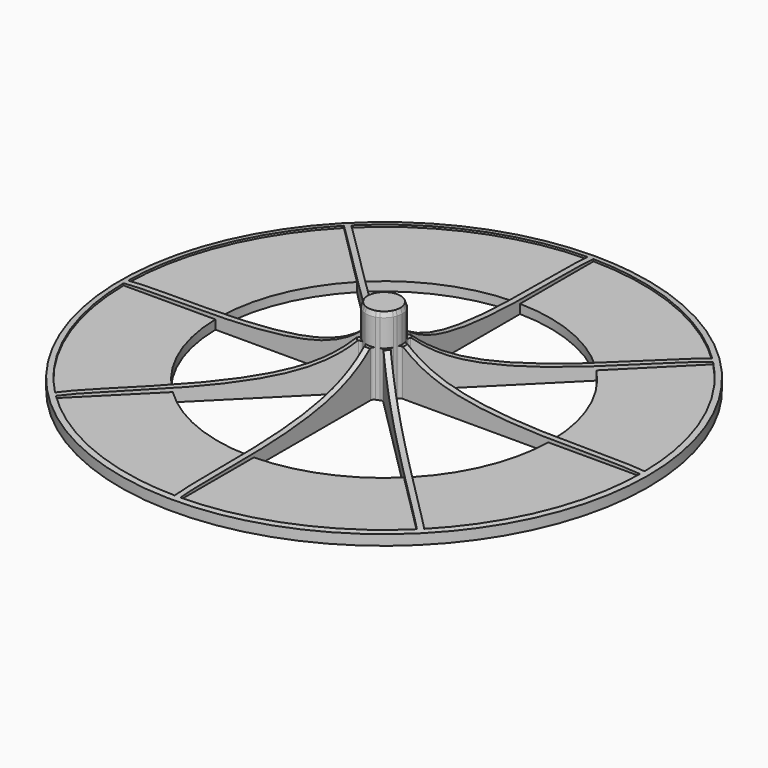
from build123d import *

# Parameters (mm, degrees)
F0_R     = 58.42
F1_DEPTH = 10.16
F2_R     = 58.42
F2_R_2   = 36.83
F3_DEPTH = 2
F7_DEPTH = 7
F8_SIZE2 = 1.0467888968
F8_SIZE  = 0.381


# Not quite as in the source:
# - a feature names something its author has since deleted; it is built from what else it names


with BuildPart() as f1:
    # F0 (on Top) → F1 (new body)
    with BuildSketch(Plane.XY):
        Circle(F0_R)
        with BuildLine():
            ThreePointArc((-0.635, -57.1464721133), (-21.8703581597, -52.799715283), (-39.9596451462, -40.8576707583))
            Line((-39.9596451462, -40.8576707583), (-27.3861598627, -28.2841854748))
            Line((-27.3861598627, -28.2841854748), (-2.7700736327, -3.6680992448))
            ThreePointArc((-2.7700736327, -3.6680992448), (-2.3442801324, -3.4533430776), (-1.8742194586, -3.5337375994))
            ThreePointArc((-1.8742194586, -3.5337375994), (-1.5307337295, -3.69551813), (-1.1734565309, -3.824003108))
            ThreePointArc((-1.1734565309, -3.824003108), (-0.7842259293, -4.0995386865), (-0.635, -4.5524757001))
            Line((-0.635, -4.5524757001), (-0.635, -38.0947079658))
            Line((-0.635, -38.0947079658), (-0.635, -57.1464721133))
        make_face(mode=Mode.SUBTRACT)
        with BuildLine():
            ThreePointArc((-40.8576707583, -39.9596451462), (-52.799715283, -21.8703581597), (-57.1464721133, -0.635))
            Line((-57.1464721133, -0.635), (-39.3648786992, -0.635))
            Line((-39.3648786992, -0.635), (-4.5524757001, -0.635))
            ThreePointArc((-4.5524757001, -0.635), (-4.0995386865, -0.7842259293), (-3.824003108, -1.1734565309))
            ThreePointArc((-3.824003108, -1.1734565309), (-3.69551813, -1.5307337295), (-3.5337375994, -1.8742194586))
            ThreePointArc((-3.5337375994, -1.8742194586), (-3.4533430776, -2.3442801324), (-3.6680992448, -2.7700736327))
            Line((-3.6680992448, -2.7700736327), (-27.386039136, -26.4880135239))
            Line((-27.386039136, -26.4880135239), (-40.8576707583, -39.9596451462))
        make_face(mode=Mode.SUBTRACT)
        with BuildLine():
            ThreePointArc((39.9596451462, -40.8576707583), (21.8703581597, -52.799715283), (0.635, -57.1464721133))
            Line((0.635, -57.1464721133), (0.635, -39.3648786992))
            Line((0.635, -39.3648786992), (0.635, -4.5524757001))
            ThreePointArc((0.635, -4.5524757001), (0.7842259293, -4.0995386865), (1.1734565309, -3.824003108))
            ThreePointArc((1.1734565309, -3.824003108), (1.5307337295, -3.69551813), (1.8742194586, -3.5337375994))
            ThreePointArc((1.8742194586, -3.5337375994), (2.3442801324, -3.4533430776), (2.7700736327, -3.6680992448))
            Line((2.7700736327, -3.6680992448), (27.3861598627, -28.2841854748))
            Line((27.3861598627, -28.2841854748), (39.9596451462, -40.8576707583))
        make_face(mode=Mode.SUBTRACT)
        with BuildLine():
            ThreePointArc((57.1464721133, -0.635), (52.799715283, -21.8703581597), (40.8576707583, -39.9596451462))
            Line((40.8576707583, -39.9596451462), (27.386039136, -26.4880135239))
            Line((27.386039136, -26.4880135239), (3.6680992448, -2.7700736327))
            ThreePointArc((3.6680992448, -2.7700736327), (3.4533430776, -2.3442801324), (3.5337375994, -1.8742194586))
            ThreePointArc((3.5337375994, -1.8742194586), (3.69551813, -1.5307337295), (3.824003108, -1.1734565309))
            ThreePointArc((3.824003108, -1.1734565309), (4.0995386865, -0.7842259293), (4.5524757001, -0.635))
            Line((4.5524757001, -0.635), (38.0947079658, -0.635))
            Line((38.0947079658, -0.635), (57.1464721133, -0.635))
        make_face(mode=Mode.SUBTRACT)
        with BuildLine():
            ThreePointArc((-3.6680992448, 2.7700736327), (-3.4533430776, 2.3442801324), (-3.5337375994, 1.8742194586))
            ThreePointArc((-3.5337375994, 1.8742194586), (-3.69551813, 1.5307337295), (-3.824003108, 1.1734565309))
            ThreePointArc((-3.824003108, 1.1734565309), (-4.0995386865, 0.7842259293), (-4.5524757001, 0.635))
            Line((-4.5524757001, 0.635), (-38.0947079658, 0.635))
            Line((-38.0947079658, 0.635), (-57.1464721133, 0.635))
            ThreePointArc((-57.1464721133, 0.635), (-52.799715283, 21.8703581597), (-40.8576707583, 39.9596451462))
            Line((-40.8576707583, 39.9596451462), (-27.386039136, 26.4880135239))
            Line((-27.386039136, 26.4880135239), (-3.6680992448, 2.7700736327))
        make_face(mode=Mode.SUBTRACT)
        with BuildLine():
            ThreePointArc((-39.9596451462, 40.8576707583), (-21.8703581597, 52.799715283), (-0.635, 57.1464721133))
            Line((-0.635, 57.1464721133), (-0.635, 39.3648786992))
            Line((-0.635, 39.3648786992), (-0.635, 4.5524757001))
            ThreePointArc((-0.635, 4.5524757001), (-0.7842259293, 4.0995386865), (-1.1734565309, 3.824003108))
            ThreePointArc((-1.1734565309, 3.824003108), (-1.5307337295, 3.69551813), (-1.8742194586, 3.5337375994))
            ThreePointArc((-1.8742194586, 3.5337375994), (-2.3442801324, 3.4533430776), (-2.7700736327, 3.6680992448))
            Line((-2.7700736327, 3.6680992448), (-26.4880135239, 27.386039136))
            Line((-26.4880135239, 27.386039136), (-39.9596451462, 40.8576707583))
        make_face(mode=Mode.SUBTRACT)
        with BuildLine():
            ThreePointArc((40.8576707583, 39.9596451462), (52.799715283, 21.8703581597), (57.1464721133, 0.635))
            Line((57.1464721133, 0.635), (39.3648786992, 0.635))
            Line((39.3648786992, 0.635), (4.5524757001, 0.635))
            ThreePointArc((4.5524757001, 0.635), (4.0995386865, 0.7842259293), (3.824003108, 1.1734565309))
            ThreePointArc((3.824003108, 1.1734565309), (3.69551813, 1.5307337295), (3.5337375994, 1.8742194586))
            ThreePointArc((3.5337375994, 1.8742194586), (3.4533430776, 2.3442801324), (3.6680992448, 2.7700736327))
            Line((3.6680992448, 2.7700736327), (28.2841854748, 27.3861598627))
            Line((28.2841854748, 27.3861598627), (40.8576707583, 39.9596451462))
        make_face(mode=Mode.SUBTRACT)
        with BuildLine():
            Line((0.635, 38.0947079658), (0.635, 57.1464721133))
            ThreePointArc((0.635, 57.1464721133), (21.8703581597, 52.799715283), (39.9596451462, 40.8576707583))
            Line((39.9596451462, 40.8576707583), (26.4880135239, 27.386039136))
            Line((26.4880135239, 27.386039136), (2.7700736327, 3.6680992448))
            ThreePointArc((2.7700736327, 3.6680992448), (2.3442801324, 3.4533430776), (1.8742194586, 3.5337375994))
            ThreePointArc((1.8742194586, 3.5337375994), (1.5307337295, 3.69551813), (1.1734565309, 3.824003108))
            ThreePointArc((1.1734565309, 3.824003108), (0.7842259293, 4.0995386865), (0.635, 4.5524757001))
            Line((0.635, 4.5524757001), (0.635, 38.0947079658))
        make_face(mode=Mode.SUBTRACT)
    extrude(amount=F1_DEPTH)

    # F2 (on Top) → F3 (join)
    with BuildSketch(Plane.XY):
        Circle(F2_R)
        Circle(F2_R_2, mode=Mode.SUBTRACT)
    extrude(amount=F3_DEPTH)

    # F4 (on Right) → F5 (revolve, cut)
    with BuildSketch(Plane.YZ):
        with BuildLine():
            Line((62.3432286084, 24.0727756172), (0, 24.0727756172))
            Line((0, 24.0727756172), (0, 16.6299855337))
            add(Edge.make_bspline(
                [(0, 16.6299855337), (1.5198661401, 12.6081325684), (11.6499832075, 1.5638180555), (50.5879250499, 3.3015021067), (61.8285896767, 2.1889962413), (62.3432286084, 0)],
                knots=[0, 0, 0, 0, 0.2981784655, 0.7648643815, 1, 1, 1, 1], degree=3))
            Line((62.3432286084, 0), (62.3432286084, 24.0727756172))
        make_face()
    revolve(axis=Axis((0, 0, 0), (0, 0, -1)), mode=Mode.SUBTRACT)

    # F6 (on face) → F7 (join)
    with BuildSketch(Plane.XY.offset(10.16)):
        with BuildLine():
            ThreePointArc((3.824003108, -1.1734565309), (3.9557560865, -0.5932906404), (4, 0))
            ThreePointArc((4, 0), (3.9557560865, 0.5932906404), (3.824003108, 1.1734565309))
            ThreePointArc((3.824003108, 1.1734565309), (3.69551813, 1.5307337295), (3.5337375994, 1.8742194586))
            ThreePointArc((3.5337375994, 1.8742194586), (2.8284271247, 2.8284271247), (1.8742194586, 3.5337375994))
            ThreePointArc((1.8742194586, 3.5337375994), (1.5307337295, 3.69551813), (1.1734565309, 3.824003108))
            ThreePointArc((1.1734565309, 3.824003108), (0, 4), (-1.1734565309, 3.824003108))
            ThreePointArc((-1.1734565309, 3.824003108), (-1.5307337295, 3.69551813), (-1.8742194586, 3.5337375994))
            ThreePointArc((-1.8742194586, 3.5337375994), (-2.8284271247, 2.8284271247), (-3.5337375994, 1.8742194586))
            ThreePointArc((-3.5337375994, 1.8742194586), (-3.69551813, 1.5307337295), (-3.824003108, 1.1734565309))
            ThreePointArc((-3.824003108, 1.1734565309), (-4, 0), (-3.824003108, -1.1734565309))
            ThreePointArc((-3.824003108, -1.1734565309), (-3.69551813, -1.5307337295), (-3.5337375994, -1.8742194586))
            ThreePointArc((-3.5337375994, -1.8742194586), (-2.8284271247, -2.8284271247), (-1.8742194586, -3.5337375994))
            ThreePointArc((-1.8742194586, -3.5337375994), (-1.5307337295, -3.69551813), (-1.1734565309, -3.824003108))
            ThreePointArc((-1.1734565309, -3.824003108), (0, -4), (1.1734565309, -3.824003108))
            ThreePointArc((1.1734565309, -3.824003108), (1.5307337295, -3.69551813), (1.8742194586, -3.5337375994))
            ThreePointArc((1.8742194586, -3.5337375994), (2.8284271247, -2.8284271247), (3.5337375994, -1.8742194586))
            ThreePointArc((3.5337375994, -1.8742194586), (3.69551813, -1.5307337295), (3.824003108, -1.1734565309))
        make_face()
    extrude(amount=F7_DEPTH)

    # F8
    f8_edges = [f1.edges().sort_by_distance(p)[0] for p in [
        (-3.533738, 1.874219, 17.16),
    ]]
    f8_side = f1.faces().sort_by_distance((0, 0, 17.16))[0]
    chamfer(f8_edges, length=F8_SIZE, length2=F8_SIZE2, reference=f8_side)


solid = f1.part
